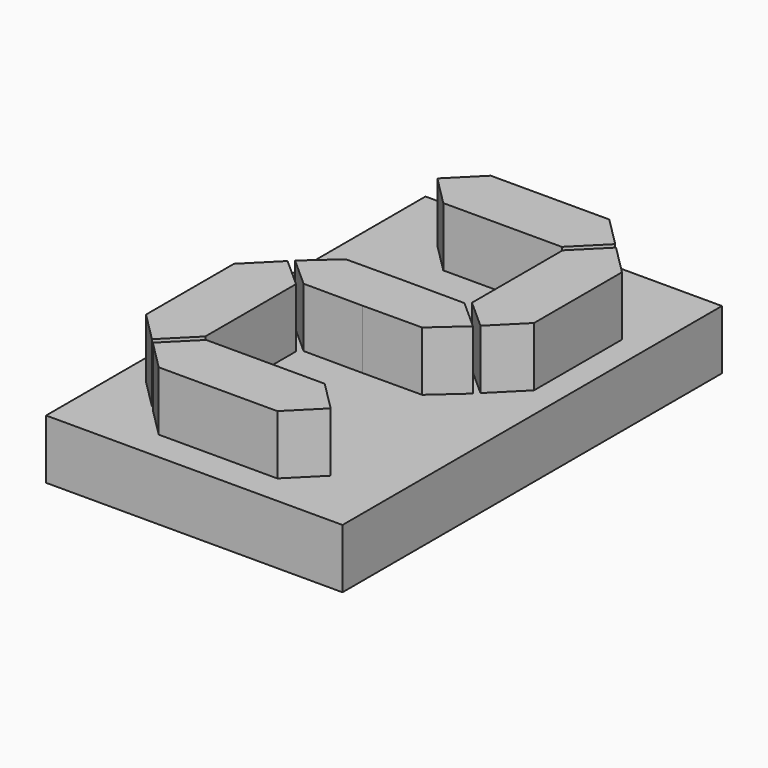
from build123d import *

# Parameters (mm, degrees)
F0_W     = 10
F0_H     = 16
F1_DEPTH = 2
F3_DEPTH = 2


# Not quite as in the source:
# - ends of sketch curves that miss each other by under 0.0002 mm in the source are joined


with BuildPart() as f1:
    # F0 (on Top) → F1 (new body)
    with BuildSketch(Plane.XY):
        Rectangle(F0_W, F0_H)
    extrude(amount=F1_DEPTH)

    # F2 (on face) → F3 (join)
    with BuildSketch(Plane.XY.offset(2)):
        Polygon((0, 7), (-2, 7), (-3, 6), (-2, 5), (0, 5), (2, 5), (3, 6), (2, 7), align=None)
        Polygon((2, 0.891659756), (2.00782e-05, 0.9006214721), (-2, 0.891659756), (-3, 0), (-2, -0.891659756), (-2.00782e-05, -0.9006214721), (2, -0.891659756), (3, 0), align=None)
        Polygon((0, -5), (-2, -5), (-3, -6), (-2, -7), (0, -7), (2, -7), (3, -6), (2, -5), align=None)
        Polygon((-4.1414213562, -4.8585786438), (-3.1414213562, -5.8585786438), (-2.1414213562, -4.8585786438), (-2.1414213562, -1.0335195075), (-3.1374518146, -0.1453992321), (-4.1414213562, -1.1507223826), align=None)
        Polygon((4.1414213562, 4.8585786438), (3.1414213562, 5.8585786438), (2.1414213562, 4.8585786438), (2.1414213562, 1.0335195075), (3.1374518146, 0.1453992321), (4.1414213562, 1.1507223826), align=None)
    extrude(amount=F3_DEPTH)


solid = f1.part
